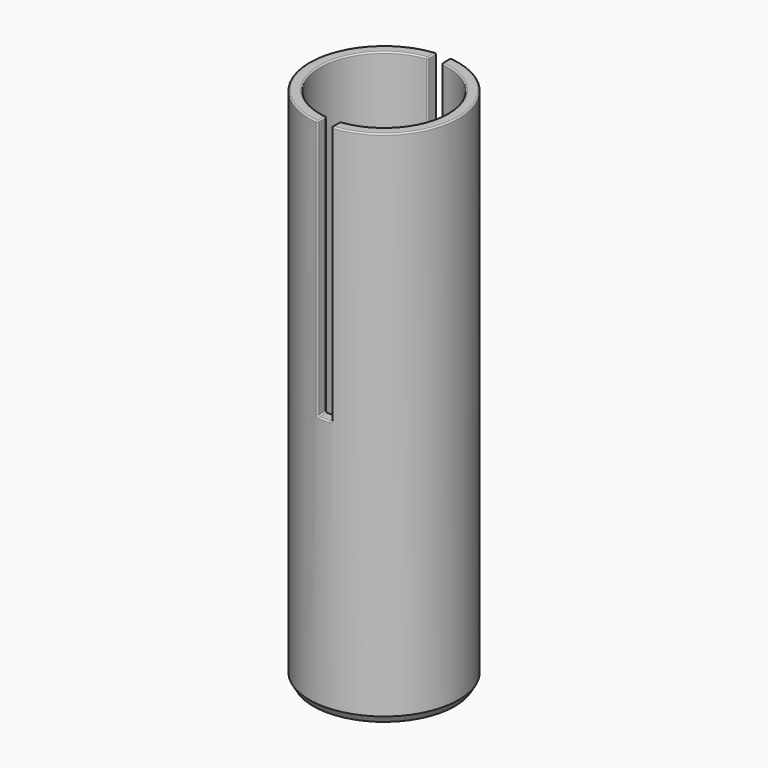
from build123d import *

# Parameters (mm, degrees)
F0_R     = 5.48
F1_DEPTH = 38.1
F2_T     = -0.8
F4_DEPTH = 19.05
F5_F1_R  = 0.100000054
F5_F2_R  = 0.100000054
F6_SIZE2 = 0.2886751346
F6_SIZE  = 0.5


with BuildPart() as f1:
    # F0 (on Top) → F1 (new body)
    with BuildSketch(Plane.XY):
        Circle(F0_R)
    extrude(amount=F1_DEPTH)

    # F2
    f2_openings = [f1.faces().sort_by_distance(p)[0] for p in [
        (0, 0, 38.1),
    ]]
    offset(amount=F2_T, openings=f2_openings)

    # F3 (on face) → F4 (cut)
    with BuildSketch(Plane.XY.offset(38.1)):
        with BuildLine():
            Line((0.508, 4.6523473645), (0.508, 5.4564032109))
            ThreePointArc((0.508, 5.4564032109), (0, 5.48), (-0.508, 5.4564032109))
            Line((-0.508, 5.4564032109), (-0.508, 4.6523473645))
            ThreePointArc((-0.508, 4.6523473645), (0, 4.68), (0.508, 4.6523473645))
        make_face()
        with BuildLine():
            Line((0.508, -5.4564032109), (0.508, -4.6523473645))
            ThreePointArc((0.508, -4.6523473645), (0, -4.68), (-0.508, -4.6523473645))
            Line((-0.508, -4.6523473645), (-0.508, -5.4564032109))
            ThreePointArc((-0.508, -5.4564032109), (0, -5.48), (0.508, -5.4564032109))
        make_face()
    extrude(amount=-F4_DEPTH, mode=Mode.SUBTRACT)

    # F5: fillet of radius 0.100000054 on 20 edges, made by hand

    # F5_f1
    f5_f1_edges = [f1.edges().sort_by_distance(p)[0] for p in [
        (0.508, -5.0543752877, 19.05),
        (-0.508, -5.0543752877, 19.05),
        (-0.508, 5.0543752877, 19.05),
        (0.508, 5.0543752877, 19.05),
    ]]
    fillet(f5_f1_edges, radius=F5_F1_R)

    # F5_f2
    f5_f2_edges = [f1.edges().sort_by_distance(p)[0] for p in [
        (-0.508, 5.0543752877, 38.1),
        (-4.68, 0, 38.1),
        (-0.508, -5.0543752877, 38.1),
        (-5.48, 0, 38.1),
        (4.0505703302, -3.6909727715, 38.1),
        (0.508, -5.0543752877, 38.1),
        (3.4842387978, -3.1244967595, 38.1),
        (3.4842387978, 3.1244967595, 38.1),
        (0.508, 5.0543752877, 38.1),
        (4.0505703302, 3.6909727715, 38.1),
        (0.508, -5.4564032109, 28.625000027),
        (0.508, -4.6523473645, 28.625000027),
        (-0.508, -4.6523473645, 28.625000027),
        (-0.508, -5.4564032109, 28.625000027),
        (0, 4.68, 19.05),
        (0, 5.48, 19.05),
        (0.4787933813, 5.4590435891, 19.0793721529),
        (-0.4787933846, 5.4590435887, 19.0793721564),
        (-0.4787918965, 4.6554439453, 19.0793706648),
        (0.4787918943, 4.6554439457, 19.0793706623),
        (-0.4787933813, -5.4590435891, 19.0793721529),
        (-0.4787918943, -4.6554439457, 19.0793706623),
        (0.4787918943, -4.6554439457, 19.0793706623),
        (0.4787933813, -5.4590435891, 19.0793721529),
    ]]
    fillet(f5_f2_edges, radius=F5_F2_R)

    # F6
    f6_edges = [f1.edges().sort_by_distance(p)[0] for p in [
        (-5.48, 0, 0),
    ]]
    f6_side = f1.faces().sort_by_distance((-5.48, 0, 19))[0]
    chamfer(f6_edges, length=F6_SIZE, length2=F6_SIZE2, reference=f6_side)


solid = f1.part
